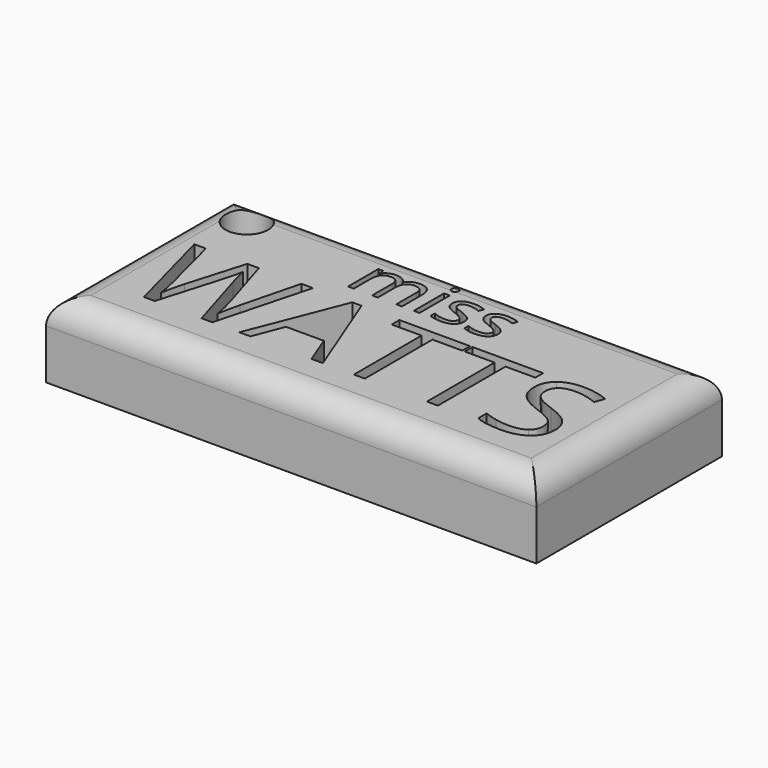
from build123d import *

# Parameters (mm, degrees)
F0_W        = 98.5645540059
F0_H        = 46.6380780563
F0_R        = 4.2775353983
F0_W_2      = 1.1529208568
F0_H_2      = 7.6083890841
F1_DEPTH    = 15
F2_T1_DEPTH = 123.5645540059
F2_T3_DEPTH = 71.6380780563


# Not quite as in the source:
# - a fillet or chamfer that OpenCascade refuses, or shapes differently, is made with other operations: its cross-section is extruded or revolved along the edge and cut away or added


with BuildPart() as f1:
    # F0 (on Top) → F1 (new body)
    with BuildSketch(Plane.XY):
        with Locations((-6.359456107, 10.058328975)):
            Rectangle(F0_W, F0_H)
        with BuildLine():
            Line((-24.9625813412, 15.4574157186), (-30.0306754022, -3.4919474274))
            Line((-30.0306754022, -3.4919474274), (-32.2080480552, -3.4919474274))
            Line((-32.2080480552, -3.4919474274), (-36.0319291716, 9.1948772309))
            add(Edge.make_bspline(
                [(-36.0319291716, 9.1948772309), (-36.3056560194, 10.0409420332), (-36.6415935144, 11.3224813661)],
                knots=[0, 0, 0, 1, 1, 1], degree=2))
            add(Edge.make_bspline(
                [(-36.6415935144, 11.3224813661), (-36.9775310094, 12.604020699), (-36.9899731389, 12.8653054174)],
                knots=[0, 0, 0, 1, 1, 1], degree=2))
            add(Edge.make_bspline(
                [(-36.9899731389, 12.8653054174), (-37.2761421161, 11.1524389304), (-37.8982485884, 9.1202244542)],
                knots=[0, 0, 0, 1, 1, 1], degree=2))
            Line((-37.8982485884, 9.1202244542), (-41.6060031633, -3.4919474274))
            Line((-41.6060031633, -3.4919474274), (-43.7833758163, -3.4919474274))
            Line((-43.7833758163, -3.4919474274), (-48.8265856184, 15.4574157186))
            Line((-48.8265856184, 15.4574157186), (-46.491612659, 15.4574157186))
            Line((-46.491612659, 15.4574157186), (-43.4972068391, 3.7535192866))
            add(Edge.make_bspline(
                [(-43.4972068391, 3.7535192866), (-42.8751003668, 1.2899776563), (-42.5889313895, -0.7049104315)],
                knots=[0, 0, 0, 1, 1, 1], degree=2))
            add(Edge.make_bspline(
                [(-42.5889313895, -0.7049104315), (-42.240551765, 1.6673889162), (-41.552087269, 3.9360038518)],
                knots=[0, 0, 0, 1, 1, 1], degree=2))
            Line((-41.552087269, 3.9360038518), (-38.1595333068, 15.4574157186))
            Line((-38.1595333068, 15.4574157186), (-35.8245603475, 15.4574157186))
            Line((-35.8245603475, 15.4574157186), (-32.2619639495, 3.8323194397))
            add(Edge.make_bspline(
                [(-32.2619639495, 3.8323194397), (-31.6398574772, 1.820841846), (-31.2126776995, -0.7049104315)],
                knots=[0, 0, 0, 1, 1, 1], degree=2))
            add(Edge.make_bspline(
                [(-31.2126776995, -0.7049104315), (-30.9638351106, 1.1365247265), (-30.2795179911, 3.7784035455)],
                knots=[0, 0, 0, 1, 1, 1], degree=2))
            Line((-30.2795179911, 3.7784035455), (-27.2975543006, 15.4574157186))
            Line((-27.2975543006, 15.4574157186), (-24.9625813412, 15.4574157186))
        make_face(mode=Mode.SUBTRACT)
        Polygon((-7.8048848354, -3.4919474274), (-10.0859419005, -3.4919474274), (-12.4457991187, 2.5341906009), (-20.0396454572, 2.5341906009), (-22.37047104, -3.4919474274), (-24.6017595873, -3.4919474274), (-17.1115976609, 15.5362158718), (-15.2577203735, 15.5362158718), align=None, mode=Mode.SUBTRACT)
        Polygon((0.6308789289, 13.4998540191), (0.6308789289, -3.4919474274), (-1.5713779831, -3.4919474274), (-1.5713779831, 13.4998540191), (-7.5726317524, 13.4998540191), (-7.5726317524, 15.4574157186), (6.6321326982, 15.4574157186), (6.6321326982, 13.4998540191), align=None, mode=Mode.SUBTRACT)
        Polygon((15.3167390514, 13.4998540191), (15.3167390514, -3.4919474274), (13.1144821395, -3.4919474274), (13.1144821395, 13.4998540191), (7.1132283701, 13.4998540191), (7.1132283701, 15.4574157186), (21.3179928208, 15.4574157186), (21.3179928208, 13.4998540191), align=None, mode=Mode.SUBTRACT)
        with BuildLine():
            add(Edge.make_bspline(
                [(33.7435327607, 4.7115632539), (34.8633244109, 3.4922345682), (34.8633244109, 1.5512623747)],
                knots=[0, 0, 0, 1, 1, 1], degree=2))
            add(Edge.make_bspline(
                [(34.8633244109, 1.5512623747), (34.8633244109, -0.949605644), (33.0488472, -2.3514188949)],
                knots=[0, 0, 0, 1, 1, 1], degree=2))
            add(Edge.make_bspline(
                [(33.0488472, -2.3514188949), (31.2343699892, -3.7532321458), (28.1238376277, -3.7532321458)],
                knots=[0, 0, 0, 1, 1, 1], degree=2))
            add(Edge.make_bspline(
                [(28.1238376277, -3.7532321458), (24.7561679244, -3.7532321458), (22.9396170253, -2.8822830845)],
                knots=[0, 0, 0, 1, 1, 1], degree=2))
            Line((22.9396170253, -2.8822830845), (22.9396170253, -0.7588263258))
            add(Edge.make_bspline(
                [(22.9396170253, -0.7588263258), (24.1091771932, -1.2482167507), (25.4819588087, -1.5343857279)],
                knots=[0, 0, 0, 1, 1, 1], degree=2))
            add(Edge.make_bspline(
                [(25.4819588087, -1.5343857279), (26.8547404242, -1.8205547052), (28.2026377809, -1.8205547052)],
                knots=[0, 0, 0, 1, 1, 1], degree=2))
            add(Edge.make_bspline(
                [(28.2026377809, -1.8205547052), (30.4048946928, -1.8205547052), (31.5205389664, -0.9848583441)],
                knots=[0, 0, 0, 1, 1, 1], degree=2))
            add(Edge.make_bspline(
                [(31.5205389664, -0.9848583441), (32.6361832401, -0.1491619829), (32.6361832401, 1.3438935506)],
                knots=[0, 0, 0, 1, 1, 1], degree=2))
            add(Edge.make_bspline(
                [(32.6361832401, 1.3438935506), (32.6361832401, 2.3268217768), (32.240108786, 2.9551493138)],
                knots=[0, 0, 0, 1, 1, 1], degree=2))
            add(Edge.make_bspline(
                [(32.240108786, 2.9551493138), (31.844034332, 3.5834768508), (30.9170956883, 4.1164147287)],
                knots=[0, 0, 0, 1, 1, 1], degree=2))
            add(Edge.make_bspline(
                [(30.9170956883, 4.1164147287), (29.9901570446, 4.6493526067), (28.0989533688, 5.3212275967)],
                knots=[0, 0, 0, 1, 1, 1], degree=2))
            add(Edge.make_bspline(
                [(28.0989533688, 5.3212275967), (25.4570745498, 6.2668294346), (24.322767082, 7.5628845852)],
                knots=[0, 0, 0, 1, 1, 1], degree=2))
            add(Edge.make_bspline(
                [(24.322767082, 7.5628845852), (23.1884596142, 8.8589397358), (23.1884596142, 10.9450701063)],
                knots=[0, 0, 0, 1, 1, 1], degree=2))
            add(Edge.make_bspline(
                [(23.1884596142, 10.9450701063), (23.1884596142, 13.1348848887), (24.8328943893, 14.4309400393)],
                knots=[0, 0, 0, 1, 1, 1], degree=2))
            add(Edge.make_bspline(
                [(24.8328943893, 14.4309400393), (26.4773291644, 15.72699519), (29.1897133836, 15.72699519)],
                knots=[0, 0, 0, 1, 1, 1], degree=2))
            add(Edge.make_bspline(
                [(29.1897133836, 15.72699519), (32.0140767678, 15.72699519), (34.3863761154, 14.6901510695)],
                knots=[0, 0, 0, 1, 1, 1], degree=2))
            Line((34.3863761154, 14.6901510695), (33.6979116194, 12.7740631348))
            add(Edge.make_bspline(
                [(33.6979116194, 12.7740631348), (31.3504965306, 13.756991361), (29.1357974893, 13.756991361)],
                knots=[0, 0, 0, 1, 1, 1], degree=2))
            add(Edge.make_bspline(
                [(29.1357974893, 13.756991361), (27.3856046139, 13.756991361), (26.4006026994, 13.0063162178)],
                knots=[0, 0, 0, 1, 1, 1], degree=2))
            add(Edge.make_bspline(
                [(26.4006026994, 13.0063162178), (25.415600785, 12.2556410746), (25.415600785, 10.9201858474)],
                knots=[0, 0, 0, 1, 1, 1], degree=2))
            add(Edge.make_bspline(
                [(25.415600785, 10.9201858474), (25.415600785, 9.9372576212), (25.7784962272, 9.3068563959)],
                knots=[0, 0, 0, 1, 1, 1], degree=2))
            add(Edge.make_bspline(
                [(25.7784962272, 9.3068563959), (26.1413916693, 8.6764551706), (27.0040459776, 8.1518120457)],
                knots=[0, 0, 0, 1, 1, 1], degree=2))
            add(Edge.make_bspline(
                [(27.0040459776, 8.1518120457), (27.8667002858, 7.6271689207), (29.6417774201, 6.992620319)],
                knots=[0, 0, 0, 1, 1, 1], degree=2))
            add(Edge.make_bspline(
                [(29.6417774201, 6.992620319), (32.6237411106, 5.9308919396), (33.7435327607, 4.7115632539)],
                knots=[0, 0, 0, 1, 1, 1], degree=2))
        make_face(mode=Mode.SUBTRACT)
        with Locations((-47.1104159951, 26.5214201063)):
            Circle(F0_R, mode=Mode.SUBTRACT)
        with BuildLine():
            Line((-10.1462676927, 19.3094518036), (-11.2969671221, 19.3094518036))
            Line((-11.2969671221, 19.3094518036), (-11.2969671221, 24.2587922063))
            add(Edge.make_bspline(
                [(-11.2969671221, 24.2587922063), (-11.2969671221, 25.169577469), (-11.6857169293, 25.6238593865)],
                knots=[0, 0, 0, 1, 1, 1], degree=2))
            add(Edge.make_bspline(
                [(-11.6857169293, 25.6238593865), (-12.0744667365, 26.0781413041), (-12.8941734729, 26.0781413041)],
                knots=[0, 0, 0, 1, 1, 1], degree=2))
            add(Edge.make_bspline(
                [(-12.8941734729, 26.0781413041), (-13.9693443683, 26.0781413041), (-14.4836048275, 25.4605844675)],
                knots=[0, 0, 0, 1, 1, 1], degree=2))
            add(Edge.make_bspline(
                [(-14.4836048275, 25.4605844675), (-14.9978652868, 24.8430276309), (-14.9978652868, 23.5590425533)],
                knots=[0, 0, 0, 1, 1, 1], degree=2))
            Line((-14.9978652868, 23.5590425533), (-14.9978652868, 19.3094518036))
            Line((-14.9978652868, 19.3094518036), (-16.1507861436, 19.3094518036))
            Line((-16.1507861436, 19.3094518036), (-16.1507861436, 24.2587922063))
            add(Edge.make_bspline(
                [(-16.1507861436, 24.2587922063), (-16.1507861436, 25.169577469), (-16.5395359509, 25.6238593865)],
                knots=[0, 0, 0, 1, 1, 1], degree=2))
            add(Edge.make_bspline(
                [(-16.5395359509, 25.6238593865), (-16.9282857581, 26.0781413041), (-17.7546567769, 26.0781413041)],
                knots=[0, 0, 0, 1, 1, 1], degree=2))
            add(Edge.make_bspline(
                [(-17.7546567769, 26.0781413041), (-18.8364919547, 26.0781413041), (-19.3396452766, 25.4294844829)],
                knots=[0, 0, 0, 1, 1, 1], degree=2))
            add(Edge.make_bspline(
                [(-19.3396452766, 25.4294844829), (-19.8427985985, 24.7808276617), (-19.8427985985, 23.3013569668)],
                knots=[0, 0, 0, 1, 1, 1], degree=2))
            Line((-19.8427985985, 23.3013569668), (-19.8427985985, 19.3094518036))
            Line((-19.8427985985, 19.3094518036), (-20.9957194553, 19.3094518036))
            Line((-20.9957194553, 19.3094518036), (-20.9957194553, 26.9178408877))
            Line((-20.9957194553, 26.9178408877), (-20.0582770631, 26.9178408877))
            Line((-20.0582770631, 26.9178408877), (-19.8716771556, 25.8759914044))
            Line((-19.8716771556, 25.8759914044), (-19.8161414689, 25.8759914044))
            add(Edge.make_bspline(
                [(-19.8161414689, 25.8759914044), (-19.4895916308, 26.4313482718), (-18.8953597826, 26.7445695451)],
                knots=[0, 0, 0, 1, 1, 1], degree=2))
            add(Edge.make_bspline(
                [(-18.8953597826, 26.7445695451), (-18.3011279344, 27.0577908183), (-17.5658354419, 27.0577908183)],
                knots=[0, 0, 0, 1, 1, 1], degree=2))
            add(Edge.make_bspline(
                [(-17.5658354419, 27.0577908183), (-15.7820291837, 27.0577908183), (-15.2333365986, 25.7649200309)],
                knots=[0, 0, 0, 1, 1, 1], degree=2))
            Line((-15.2333365986, 25.7649200309), (-15.1778009119, 25.7649200309))
            add(Edge.make_bspline(
                [(-15.1778009119, 25.7649200309), (-14.837922509, 26.3624840203), (-14.192597829, 26.7101374193)],
                knots=[0, 0, 0, 1, 1, 1], degree=2))
            add(Edge.make_bspline(
                [(-14.192597829, 26.7101374193), (-13.547273149, 27.0577908183), (-12.7209021302, 27.0577908183)],
                knots=[0, 0, 0, 1, 1, 1], degree=2))
            add(Edge.make_bspline(
                [(-12.7209021302, 27.0577908183), (-11.4302527703, 27.0577908183), (-10.7882602315, 26.3946947186)],
                knots=[0, 0, 0, 1, 1, 1], degree=2))
            add(Edge.make_bspline(
                [(-10.7882602315, 26.3946947186), (-10.1462676927, 25.7315986188), (-10.1462676927, 24.2721207712)],
                knots=[0, 0, 0, 1, 1, 1], degree=2))
            Line((-10.1462676927, 24.2721207712), (-10.1462676927, 19.3094518036))
        make_face(mode=Mode.SUBTRACT)
        with Locations((-7.1951012991, 23.1136463456)):
            Rectangle(F0_W_2, F0_H_2, mode=Mode.SUBTRACT)
        with BuildLine():
            add(Edge.make_bspline(
                [(-7.6749296325, 28.3995330101), (-7.8693045361, 28.5905757725), (-7.8693045361, 28.9793255797)],
                knots=[0, 0, 0, 1, 1, 1], degree=2))
            add(Edge.make_bspline(
                [(-7.8693045361, 28.9793255797), (-7.8693045361, 29.3747396693), (-7.6749296325, 29.5591181493)],
                knots=[0, 0, 0, 1, 1, 1], degree=2))
            add(Edge.make_bspline(
                [(-7.6749296325, 29.5591181493), (-7.4805547289, 29.7434966293), (-7.1873263029, 29.7434966293)],
                knots=[0, 0, 0, 1, 1, 1], degree=2))
            add(Edge.make_bspline(
                [(-7.1873263029, 29.7434966293), (-6.9096478692, 29.7434966293), (-6.7086086832, 29.5557860081)],
                knots=[0, 0, 0, 1, 1, 1], degree=2))
            add(Edge.make_bspline(
                [(-6.7086086832, 29.5557860081), (-6.5075694971, 29.3680753869), (-6.5075694971, 28.9793255797)],
                knots=[0, 0, 0, 1, 1, 1], degree=2))
            add(Edge.make_bspline(
                [(-6.5075694971, 28.9793255797), (-6.5075694971, 28.5905757725), (-6.7086086832, 28.3995330101)],
                knots=[0, 0, 0, 1, 1, 1], degree=2))
            add(Edge.make_bspline(
                [(-6.7086086832, 28.3995330101), (-6.9096478692, 28.2084902477), (-7.1873263029, 28.2084902477)],
                knots=[0, 0, 0, 1, 1, 1], degree=2))
            add(Edge.make_bspline(
                [(-7.1873263029, 28.2084902477), (-7.4805547289, 28.2084902477), (-7.6749296325, 28.3995330101)],
                knots=[0, 0, 0, 1, 1, 1], degree=2))
        make_face(mode=Mode.SUBTRACT)
        with BuildLine():
            add(Edge.make_bspline(
                [(0.2566771485, 22.6415930083), (0.732062627, 22.1417718276), (0.732062627, 21.3842650604)],
                knots=[0, 0, 0, 1, 1, 1], degree=2))
            add(Edge.make_bspline(
                [(0.732062627, 21.3842650604), (0.732062627, 20.3224227298), (-0.0587655522, 19.7459623014)],
                knots=[0, 0, 0, 1, 1, 1], degree=2))
            add(Edge.make_bspline(
                [(-0.0587655522, 19.7459623014), (-0.8495937315, 19.169501873), (-2.2801930221, 19.169501873)],
                knots=[0, 0, 0, 1, 1, 1], degree=2))
            add(Edge.make_bspline(
                [(-2.2801930221, 19.169501873), (-3.792985129, 19.169501873), (-4.639348995, 19.6493302064)],
                knots=[0, 0, 0, 1, 1, 1], degree=2))
            Line((-4.639348995, 19.6493302064), (-4.639348995, 20.7178368194))
            add(Edge.make_bspline(
                [(-4.639348995, 20.7178368194), (-4.09065641, 20.4401583857), (-3.4631031497, 20.2813263216)],
                knots=[0, 0, 0, 1, 1, 1], degree=2))
            add(Edge.make_bspline(
                [(-3.4631031497, 20.2813263216), (-2.8355498895, 20.1224942575), (-2.251314465, 20.1224942575)],
                knots=[0, 0, 0, 1, 1, 1], degree=2))
            add(Edge.make_bspline(
                [(-2.251314465, 20.1224942575), (-1.3494149122, 20.1224942575), (-0.8640330101, 20.4101691149)],
                knots=[0, 0, 0, 1, 1, 1], degree=2))
            add(Edge.make_bspline(
                [(-0.8640330101, 20.4101691149), (-0.3786511079, 20.6978439722), (-0.3786511079, 21.2887436792)],
                knots=[0, 0, 0, 1, 1, 1], degree=2))
            add(Edge.make_bspline(
                [(-0.3786511079, 21.2887436792), (-0.3786511079, 21.7330291731), (-0.7629580602, 22.0484718739)],
                knots=[0, 0, 0, 1, 1, 1], degree=2))
            add(Edge.make_bspline(
                [(-0.7629580602, 22.0484718739), (-1.1472650125, 22.3639145746), (-2.2668644572, 22.7948715037)],
                knots=[0, 0, 0, 1, 1, 1], degree=2))
            add(Edge.make_bspline(
                [(-2.2668644572, 22.7948715037), (-3.3287067878, 23.1902855933), (-3.776324423, 23.4857354468)],
                knots=[0, 0, 0, 1, 1, 1], degree=2))
            add(Edge.make_bspline(
                [(-3.776324423, 23.4857354468), (-4.2239420582, 23.7811853003), (-4.4427526639, 24.155495829)],
                knots=[0, 0, 0, 1, 1, 1], degree=2))
            add(Edge.make_bspline(
                [(-4.4427526639, 24.155495829), (-4.6615632697, 24.5298063577), (-4.6615632697, 25.0496203856)],
                knots=[0, 0, 0, 1, 1, 1], degree=2))
            add(Edge.make_bspline(
                [(-4.6615632697, 25.0496203856), (-4.6615632697, 25.9803984954), (-3.9040565025, 26.5190946569)],
                knots=[0, 0, 0, 1, 1, 1], degree=2))
            add(Edge.make_bspline(
                [(-3.9040565025, 26.5190946569), (-3.1465497353, 27.0577908183), (-1.8292432457, 27.0577908183)],
                knots=[0, 0, 0, 1, 1, 1], degree=2))
            add(Edge.make_bspline(
                [(-1.8292432457, 27.0577908183), (-0.6007938549, 27.0577908183), (0.5743412767, 26.5579696376)],
                knots=[0, 0, 0, 1, 1, 1], degree=2))
            Line((0.5743412767, 26.5579696376), (0.1633771947, 25.6205272453))
            add(Edge.make_bspline(
                [(0.1633771947, 25.6205272453), (-0.9806579522, 26.0914698689), (-1.9114360621, 26.0914698689)],
                knots=[0, 0, 0, 1, 1, 1], degree=2))
            add(Edge.make_bspline(
                [(-1.9114360621, 26.0914698689), (-2.7311427984, 26.0914698689), (-3.147660449, 25.8348949962)],
                knots=[0, 0, 0, 1, 1, 1], degree=2))
            add(Edge.make_bspline(
                [(-3.147660449, 25.8348949962), (-3.5641780996, 25.5783201234), (-3.5641780996, 25.127370347)],
                knots=[0, 0, 0, 1, 1, 1], degree=2))
            add(Edge.make_bspline(
                [(-3.5641780996, 25.127370347), (-3.5641780996, 24.8208133562), (-3.407567463, 24.6064456054)],
                knots=[0, 0, 0, 1, 1, 1], degree=2))
            add(Edge.make_bspline(
                [(-3.407567463, 24.6064456054), (-3.2509568264, 24.3920778545), (-2.9044141411, 24.1977029509)],
                knots=[0, 0, 0, 1, 1, 1], degree=2))
            add(Edge.make_bspline(
                [(-2.9044141411, 24.1977029509), (-2.5578714558, 24.0033280473), (-1.5715576592, 23.6345710873)],
                knots=[0, 0, 0, 1, 1, 1], degree=2))
            add(Edge.make_bspline(
                [(-1.5715576592, 23.6345710873), (-0.2187083301, 23.141414189), (0.2566771485, 22.6415930083)],
                knots=[0, 0, 0, 1, 1, 1], degree=2))
        make_face(mode=Mode.SUBTRACT)
        with BuildLine():
            add(Edge.make_bspline(
                [(7.0386952139, 22.6415930083), (7.5140806924, 22.1417718276), (7.5140806924, 21.3842650604)],
                knots=[0, 0, 0, 1, 1, 1], degree=2))
            add(Edge.make_bspline(
                [(7.5140806924, 21.3842650604), (7.5140806924, 20.3224227298), (6.7232525131, 19.7459623014)],
                knots=[0, 0, 0, 1, 1, 1], degree=2))
            add(Edge.make_bspline(
                [(6.7232525131, 19.7459623014), (5.9324243339, 19.169501873), (4.5018250433, 19.169501873)],
                knots=[0, 0, 0, 1, 1, 1], degree=2))
            add(Edge.make_bspline(
                [(4.5018250433, 19.169501873), (2.9890329364, 19.169501873), (2.1426690704, 19.6493302064)],
                knots=[0, 0, 0, 1, 1, 1], degree=2))
            Line((2.1426690704, 19.6493302064), (2.1426690704, 20.7178368194))
            add(Edge.make_bspline(
                [(2.1426690704, 20.7178368194), (2.6913616554, 20.4401583857), (3.3189149156, 20.2813263216)],
                knots=[0, 0, 0, 1, 1, 1], degree=2))
            add(Edge.make_bspline(
                [(3.3189149156, 20.2813263216), (3.9464681759, 20.1224942575), (4.5307036004, 20.1224942575)],
                knots=[0, 0, 0, 1, 1, 1], degree=2))
            add(Edge.make_bspline(
                [(4.5307036004, 20.1224942575), (5.4326031532, 20.1224942575), (5.9179850553, 20.4101691149)],
                knots=[0, 0, 0, 1, 1, 1], degree=2))
            add(Edge.make_bspline(
                [(5.9179850553, 20.4101691149), (6.4033669575, 20.6978439722), (6.4033669575, 21.2887436792)],
                knots=[0, 0, 0, 1, 1, 1], degree=2))
            add(Edge.make_bspline(
                [(6.4033669575, 21.2887436792), (6.4033669575, 21.7330291731), (6.0190600052, 22.0484718739)],
                knots=[0, 0, 0, 1, 1, 1], degree=2))
            add(Edge.make_bspline(
                [(6.0190600052, 22.0484718739), (5.6347530529, 22.3639145746), (4.5151536081, 22.7948715037)],
                knots=[0, 0, 0, 1, 1, 1], degree=2))
            add(Edge.make_bspline(
                [(4.5151536081, 22.7948715037), (3.4533112776, 23.1902855933), (3.0056936424, 23.4857354468)],
                knots=[0, 0, 0, 1, 1, 1], degree=2))
            add(Edge.make_bspline(
                [(3.0056936424, 23.4857354468), (2.5580760072, 23.7811853003), (2.3392654014, 24.155495829)],
                knots=[0, 0, 0, 1, 1, 1], degree=2))
            add(Edge.make_bspline(
                [(2.3392654014, 24.155495829), (2.1204547957, 24.5298063577), (2.1204547957, 25.0496203856)],
                knots=[0, 0, 0, 1, 1, 1], degree=2))
            add(Edge.make_bspline(
                [(2.1204547957, 25.0496203856), (2.1204547957, 25.9803984954), (2.8779615629, 26.5190946569)],
                knots=[0, 0, 0, 1, 1, 1], degree=2))
            add(Edge.make_bspline(
                [(2.8779615629, 26.5190946569), (3.6354683301, 27.0577908183), (4.9527748197, 27.0577908183)],
                knots=[0, 0, 0, 1, 1, 1], degree=2))
            add(Edge.make_bspline(
                [(4.9527748197, 27.0577908183), (6.1812242105, 27.0577908183), (7.356359342, 26.5579696376)],
                knots=[0, 0, 0, 1, 1, 1], degree=2))
            Line((7.356359342, 26.5579696376), (6.9453952601, 25.6205272453))
            add(Edge.make_bspline(
                [(6.9453952601, 25.6205272453), (5.8013601132, 26.0914698689), (4.8705820033, 26.0914698689)],
                knots=[0, 0, 0, 1, 1, 1], degree=2))
            add(Edge.make_bspline(
                [(4.8705820033, 26.0914698689), (4.0508752669, 26.0914698689), (3.6343576163, 25.8348949962)],
                knots=[0, 0, 0, 1, 1, 1], degree=2))
            add(Edge.make_bspline(
                [(3.6343576163, 25.8348949962), (3.2178399658, 25.5783201234), (3.2178399658, 25.127370347)],
                knots=[0, 0, 0, 1, 1, 1], degree=2))
            add(Edge.make_bspline(
                [(3.2178399658, 25.127370347), (3.2178399658, 24.8208133562), (3.3744506024, 24.6064456054)],
                knots=[0, 0, 0, 1, 1, 1], degree=2))
            add(Edge.make_bspline(
                [(3.3744506024, 24.6064456054), (3.531061239, 24.3920778545), (3.8776039243, 24.1977029509)],
                knots=[0, 0, 0, 1, 1, 1], degree=2))
            add(Edge.make_bspline(
                [(3.8776039243, 24.1977029509), (4.2241466096, 24.0033280473), (5.2104604062, 23.6345710873)],
                knots=[0, 0, 0, 1, 1, 1], degree=2))
            add(Edge.make_bspline(
                [(5.2104604062, 23.6345710873), (6.5633097353, 23.141414189), (7.0386952139, 22.6415930083)],
                knots=[0, 0, 0, 1, 1, 1], degree=2))
        make_face(mode=Mode.SUBTRACT)
    extrude(amount=F1_DEPTH)

    # F2: fillet of radius 5 on 4 edges, made by hand

    # F2_s2 → F2_t1 (cut)
    with BuildSketch(Plane.YZ.offset(-68.14173311)):
        with BuildLine():
            ThreePointArc((33.3773680031, 10), (31.9129019091, 13.5355339059), (28.3773680031, 15))
            Line((28.3773680031, 15), (33.3773680031, 15))
            Line((33.3773680031, 15), (33.3773680031, 10))
        make_face()
        with BuildLine():
            ThreePointArc((-13.2607100531, 10), (-11.7962439591, 13.5355339059), (-8.2607100531, 15))
            Line((-8.2607100531, 15), (-13.2607100531, 15))
            Line((-13.2607100531, 15), (-13.2607100531, 10))
        make_face()
    extrude(amount=F2_T1_DEPTH, mode=Mode.SUBTRACT)

    # F2_s4 → F2_t3 (cut)
    with BuildSketch(Plane.XZ.offset(-45.8773680031)):
        with BuildLine():
            ThreePointArc((-55.64173311, 10), (-54.1772670159, 13.5355339059), (-50.64173311, 15))
            Line((-50.64173311, 15), (-55.64173311, 15))
            Line((-55.64173311, 15), (-55.64173311, 10))
        make_face()
        with BuildLine():
            ThreePointArc((42.9228208959, 10), (41.4583548018, 13.5355339059), (37.9228208959, 15))
            Line((37.9228208959, 15), (42.9228208959, 15))
            Line((42.9228208959, 15), (42.9228208959, 10))
        make_face()
    extrude(amount=F2_T3_DEPTH, mode=Mode.SUBTRACT)


solid = f1.part
